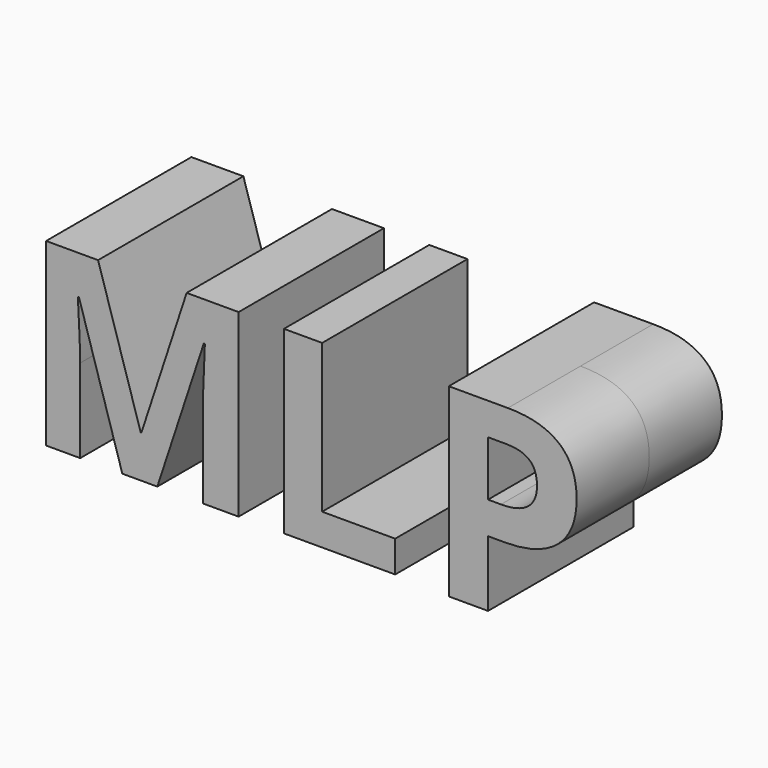
from build123d import *

# Parameters (mm, degrees)
F2_DEPTH     = 38.1
F3_TEXT_SIZE = 108.7474015852
F4_DEPTH     = 38.1


# Not quite as in the source:
# - Text() gives the source's letters only with a copy of the font that has no kerning and outlines rounded to 1/6400 em; it was checked with that copy


with BuildPart() as f2:
    # F1 (on face) + F0 (on Front) → F2 (new body, symmetric)
    with BuildSketch(Plane.XZ):
        with BuildLine():
            Line((-91.7819762693, 23.7172951289), (-91.3189554359, 23.7172951289))
            Line((-91.3189554359, 23.7172951289), (-73.1288512693, -35.5493715378))
            Line((-73.1288512693, -35.5493715378), (-58.4444762693, -35.5493715378))
            Line((-58.4444762693, -35.5493715378), (-38.9645283526, 23.6180763789))
            Line((-38.9645283526, 23.6180763789), (-38.5015075193, 23.6180763789))
            add(Edge.make_bspline(
                [(-39.1960387693, 6.0563576289), (-39.1133564776, 9.3636492956), (-38.5015075193, 23.6180763789)],
                knots=[0, 0, 0, 1, 1, 1], degree=2))
            add(Edge.make_bspline(
                [(-39.2787210609, 0.2189878372), (-39.2787210609, 2.7490659622), (-39.1960387693, 6.0563576289)],
                knots=[0, 0, 0, 1, 1, 1], degree=2))
            Line((-39.2787210609, 0.2189878372), (-39.2787210609, -35.5493715378))
            Line((-39.2787210609, -35.5493715378), (-24.3462991859, -35.5493715378))
            Line((-24.3462991859, -35.5493715378), (-24.3462991859, 40.0057065872))
            Line((-24.3462991859, 40.0057065872), (-46.1413512693, 40.0057065872))
            Line((-46.1413512693, 40.0057065872), (-65.1086689776, -17.7726788294))
            Line((-65.1086689776, -17.7726788294), (-65.4228616859, -17.7726788294))
            Line((-65.4228616859, -17.7726788294), (-83.2987731443, 40.0057065872))
            Line((-83.2987731443, 40.0057065872), (-105.1103616859, 40.0057065872))
            Line((-105.1103616859, 40.0057065872), (-105.1103616859, -35.5493715378))
            Line((-105.1103616859, -35.5493715378), (-90.7897887693, -35.5493715378))
            Line((-90.7897887693, -35.5493715378), (-90.7897887693, -0.4093975794))
            add(Edge.make_bspline(
                [(-91.7819762693, 23.7172951289), (-90.7897887693, 5.6429461706), (-90.7897887693, -0.4093975794)],
                knots=[0, 0, 0, 1, 1, 1], degree=2))
        make_face()
    with BuildSketch(Plane.XZ):
        Polygon((-5.3293721026, 40.0057065872), (-5.3293721026, -35.5493715378), (41.3365133141, -35.5493715378), (41.3365133141, -22.3202048711), (10.6944560224, -22.3202048711), (10.6944560224, 40.0057065872), align=None)
    extrude(amount=F2_DEPTH, both=True)


with BuildPart() as f4:
    # F3 (on Front) → F4 (new body, symmetric)
    with BuildSketch(Plane.XZ):
        with Locations((54.0467202663, -36.340072751)):
            Text('P', F3_TEXT_SIZE, font='Open Sans', font_style=FontStyle.BOLD, text_align=(TextAlign.LEFT, TextAlign.BOTTOM))
    extrude(amount=F4_DEPTH, both=True)


solid = Compound([f2.part, f4.part])
